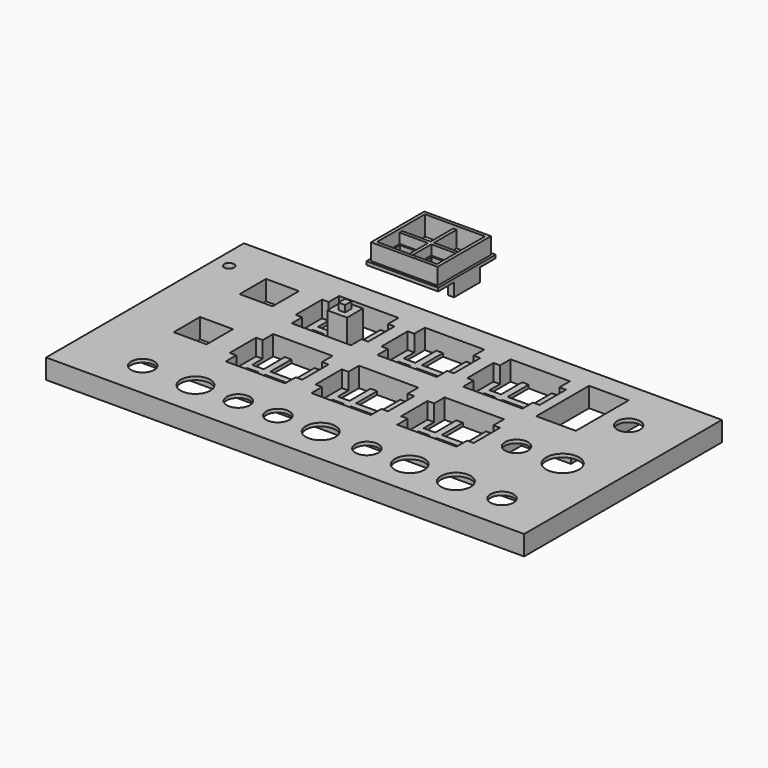
from build123d import *

# Parameters (mm, degrees)
F0_W      = 145
F0_H      = 75
F0_R      = 3.5
F0_R_2    = 4.5
F0_R_3    = 5
F0_R_4    = 1.5
F0_W_2    = 12
F0_H_2    = 20
F0_W_3    = 2
F0_H_3    = 10
F1_DEPTH  = 1
F2_DEPTH  = 5
F3_W      = 2
F3_H      = 10
F3_W_2    = 10
F4_DEPTH  = 5
F5_W      = 1.8
F5_H      = 9.8
F6_DEPTH  = 1
F7_DEPTH  = 4
F8_W      = 20.2
F8_H      = 20.2
F8_W_2    = 18.2
F8_H_2    = 18.2
F9_DEPTH  = 5
F11_W     = 6
F11_H     = 4
F11_H_2   = 2
F12_DEPTH = 8
F10_W     = 8.6
F10_H     = 1
F10_W_2   = 1
F10_H_2   = 8.6
F13_DEPTH = 6
F14_W     = 18.2
F14_H     = 18.2
F15_DEPTH = 1
F17_W     = 2
F17_H     = 2.5
F18_DEPTH = 2
F19_W     = 8.6
F19_H     = 8.6
F19_W_2   = 7.6
F19_H_2   = 7.6
F20_DEPTH = 2
F16_W     = 2
F16_H     = 2.5
F21_DEPTH = 2
F23_DEPTH = 5
F24_W     = 34
F24_H     = 2
F24_W_2   = 19
F25_DEPTH = 5


with BuildPart() as f1:
    # F0 (on Top) → F1 (new body)
    with BuildSketch(Plane.XY):
        with Locations((-82.504784634, -17.5405644029)):
            Rectangle(F0_W, F0_H)
        with Locations((-134.504784634, -44.0405644029)):
            Circle(F0_R, mode=Mode.SUBTRACT)
        with Locations((-118.504784634, -44.0405644029)):
            Circle(F0_R_2, mode=Mode.SUBTRACT)
        with Locations((-105.504784634, -44.0405644029)):
            Circle(F0_R, mode=Mode.SUBTRACT)
        with Locations((-93.504784634, -44.0405644029)):
            Circle(F0_R, mode=Mode.SUBTRACT)
        Polygon((-129.504784634, -16.0405644029), (-129.504784634, -26.0405644029), (-133.504784634, -26.0405644029), (-135.504784634, -26.0405644029), (-139.504784634, -26.0405644029), (-139.504784634, -16.0405644029), (-135.504784634, -16.0405644029), (-133.504784634, -16.0405644029), align=None, mode=Mode.SUBTRACT)
        Polygon((-102.504784634, -22.0405644029), (-102.504784634, -30.0405644029), (-105.9770819313, -30.0405644029), (-107.9770819313, -30.0405644029), (-114.9770819313, -30.0405644029), (-116.9770819313, -30.0405644029), (-120.504784634, -30.0405644029), (-120.504784634, -22.0405644029), (-120.504784634, -20.0405644029), (-120.504784634, -12.0405644029), (-116.9770819313, -12.0405644029), (-114.9770819313, -12.0405644029), (-107.9770819313, -12.0405644029), (-105.9770819313, -12.0405644029), (-102.504784634, -12.0405644029), (-102.504784634, -20.0405644029), align=None, mode=Mode.SUBTRACT)
        Polygon((-76.504784634, -12.0405644029), (-76.504784634, -20.0405644029), (-76.504784634, -22.0405644029), (-76.504784634, -30.0405644029), (-79.9770819313, -30.0405644029), (-81.9770819313, -30.0405644029), (-88.9770819313, -30.0405644029), (-90.9770819313, -30.0405644029), (-94.504784634, -30.0405644029), (-94.504784634, -22.0405644029), (-94.504784634, -20.0405644029), (-94.504784634, -12.0405644029), (-90.9770819313, -12.0405644029), (-88.9770819313, -12.0405644029), (-81.9770819313, -12.0405644029), (-79.9770819313, -12.0405644029), align=None, mode=Mode.SUBTRACT)
        with Locations((-80.504784634, -44.0405644029)):
            Circle(F0_R_2, mode=Mode.SUBTRACT)
        with Locations((-66.504784634, -44.0405644029)):
            Circle(F0_R, mode=Mode.SUBTRACT)
        with Locations((-53.504784634, -44.0405644029)):
            Circle(F0_R_2, mode=Mode.SUBTRACT)
        with Locations((-39.504784634, -44.0405644029)):
            Circle(F0_R_2, mode=Mode.SUBTRACT)
        with Locations((-25.504784634, -44.0405644029)):
            Circle(F0_R, mode=Mode.SUBTRACT)
        Polygon((-50.504784634, -12.0405644029), (-50.504784634, -20.0405644029), (-50.504784634, -22.0405644029), (-50.504784634, -30.0405644029), (-53.9770819313, -30.0405644029), (-55.9770819313, -30.0405644029), (-62.9770819313, -30.0405644029), (-64.9770819313, -30.0405644029), (-68.504784634, -30.0405644029), (-68.504784634, -22.0405644029), (-68.504784634, -20.0405644029), (-68.504784634, -12.0405644029), (-64.9770819313, -12.0405644029), (-62.9770819313, -12.0405644029), (-55.9770819313, -12.0405644029), (-53.9770819313, -12.0405644029), align=None, mode=Mode.SUBTRACT)
        with Locations((-39.504784634, -21.0405644029)):
            Circle(F0_R, mode=Mode.SUBTRACT)
        with Locations((-25.504784634, -21.0405644029)):
            Circle(F0_R_3, mode=Mode.SUBTRACT)
        with Locations((-150.504784634, 8.7571097538)):
            Circle(F0_R_4, mode=Mode.SUBTRACT)
        Polygon((-129.504784634, 8.9594355971), (-129.504784634, -1.0405644029), (-133.504784634, -1.0405644029), (-135.504784634, -1.0405644029), (-139.504784634, -1.0405644029), (-139.504784634, 8.9594355971), (-135.504784634, 8.9594355971), (-133.504784634, 8.9594355971), align=None, mode=Mode.SUBTRACT)
        Polygon((-102.504784634, 2.9594355971), (-102.504784634, -5.0405644029), (-106.004784634, -5.0405644029), (-108.004784634, -5.0405644029), (-115.004784634, -5.0405644029), (-117.004784634, -5.0405644029), (-120.504784634, -5.0405644029), (-120.504784634, 2.9594355971), (-120.504784634, 4.9594355971), (-120.504784634, 12.9594355971), (-117.004784634, 12.9594355971), (-115.004784634, 12.9594355971), (-108.004784634, 12.9594355971), (-106.004784634, 12.9594355971), (-102.504784634, 12.9594355971), (-102.504784634, 4.9594355971), align=None, mode=Mode.SUBTRACT)
        Polygon((-94.504784634, 12.9594355971), (-91.004784634, 12.9594355971), (-89.004784634, 12.9594355971), (-82.004784634, 12.9594355971), (-80.004784634, 12.9594355971), (-76.504784634, 12.9594355971), (-76.504784634, 4.9594355971), (-76.504784634, 2.9594355971), (-76.504784634, -5.0405644029), (-80.004784634, -5.0405644029), (-82.004784634, -5.0405644029), (-89.004784634, -5.0405644029), (-91.004784634, -5.0405644029), (-94.504784634, -5.0405644029), (-94.504784634, 2.9594355971), (-94.504784634, 4.9594355971), align=None, mode=Mode.SUBTRACT)
        Polygon((-68.504784634, 12.9594355971), (-65.004784634, 12.9594355971), (-63.004784634, 12.9594355971), (-56.004784634, 12.9594355971), (-54.004784634, 12.9594355971), (-50.504784634, 12.9594355971), (-50.504784634, 4.9594355971), (-50.504784634, 2.9594355971), (-50.504784634, -5.0405644029), (-54.004784634, -5.0405644029), (-56.004784634, -5.0405644029), (-63.004784634, -5.0405644029), (-65.004784634, -5.0405644029), (-68.504784634, -5.0405644029), (-68.504784634, 2.9594355971), (-68.504784634, 4.9594355971), align=None, mode=Mode.SUBTRACT)
        with Locations((-39.504784634, 3.9594355971)):
            Rectangle(F0_W_2, F0_H_2, mode=Mode.SUBTRACT)
        with Locations((-25.504784634, 3.9594355971)):
            Circle(F0_R, mode=Mode.SUBTRACT)
        Polygon((-108.004784634, -5.0405644029), (-106.004784634, -5.0405644029), (-106.004784634, 2.9594355971), (-102.504784634, 2.9594355971), (-102.504784634, 4.9594355971), (-106.004784634, 4.9594355971), (-106.004784634, 12.9594355971), (-108.004784634, 12.9594355971), (-108.004784634, 4.9594355971), (-115.004784634, 4.9594355971), (-115.004784634, 12.9594355971), (-117.004784634, 12.9594355971), (-117.004784634, 4.9594355971), (-120.504784634, 4.9594355971), (-120.504784634, 2.9594355971), (-117.004784634, 2.9594355971), (-117.004784634, -5.0405644029), (-115.004784634, -5.0405644029), (-115.004784634, 2.9594355971), (-108.004784634, 2.9594355971), align=None)
        Polygon((-107.9770819313, -30.0405644029), (-105.9770819313, -30.0405644029), (-105.9770819313, -22.0405644029), (-102.504784634, -22.0405644029), (-102.504784634, -20.0405644029), (-105.9770819313, -20.0405644029), (-105.9770819313, -12.0405644029), (-107.9770819313, -12.0405644029), (-107.9770819313, -20.0405644029), (-114.9770819313, -20.0405644029), (-114.9770819313, -12.0405644029), (-116.9770819313, -12.0405644029), (-116.9770819313, -20.0405644029), (-120.504784634, -20.0405644029), (-120.504784634, -22.0405644029), (-116.9770819313, -22.0405644029), (-116.9770819313, -30.0405644029), (-114.9770819313, -30.0405644029), (-114.9770819313, -22.0405644029), (-107.9770819313, -22.0405644029), align=None)
        Polygon((-91.004784634, 12.9594355971), (-91.004784634, 4.9594355971), (-94.504784634, 4.9594355971), (-94.504784634, 2.9594355971), (-91.004784634, 2.9594355971), (-91.004784634, -5.0405644029), (-89.004784634, -5.0405644029), (-89.004784634, 2.9594355971), (-82.004784634, 2.9594355971), (-82.004784634, -5.0405644029), (-80.004784634, -5.0405644029), (-80.004784634, 2.9594355971), (-76.504784634, 2.9594355971), (-76.504784634, 4.9594355971), (-80.004784634, 4.9594355971), (-80.004784634, 12.9594355971), (-82.004784634, 12.9594355971), (-82.004784634, 4.9594355971), (-89.004784634, 4.9594355971), (-89.004784634, 12.9594355971), align=None)
        Polygon((-65.004784634, 12.9594355971), (-65.004784634, 4.9594355971), (-68.504784634, 4.9594355971), (-68.504784634, 2.9594355971), (-65.004784634, 2.9594355971), (-65.004784634, -5.0405644029), (-63.004784634, -5.0405644029), (-63.004784634, 2.9594355971), (-56.004784634, 2.9594355971), (-56.004784634, -5.0405644029), (-54.004784634, -5.0405644029), (-54.004784634, 2.9594355971), (-50.504784634, 2.9594355971), (-50.504784634, 4.9594355971), (-54.004784634, 4.9594355971), (-54.004784634, 12.9594355971), (-56.004784634, 12.9594355971), (-56.004784634, 4.9594355971), (-63.004784634, 4.9594355971), (-63.004784634, 12.9594355971), align=None)
        Polygon((-50.504784634, -22.0405644029), (-50.504784634, -20.0405644029), (-53.9770819313, -20.0405644029), (-53.9770819313, -12.0405644029), (-55.9770819313, -12.0405644029), (-55.9770819313, -20.0405644029), (-62.9770819313, -20.0405644029), (-62.9770819313, -12.0405644029), (-64.9770819313, -12.0405644029), (-64.9770819313, -20.0405644029), (-68.504784634, -20.0405644029), (-68.504784634, -22.0405644029), (-64.9770819313, -22.0405644029), (-64.9770819313, -30.0405644029), (-62.9770819313, -30.0405644029), (-62.9770819313, -22.0405644029), (-55.9770819313, -22.0405644029), (-55.9770819313, -30.0405644029), (-53.9770819313, -30.0405644029), (-53.9770819313, -22.0405644029), align=None)
        Polygon((-76.504784634, -22.0405644029), (-76.504784634, -20.0405644029), (-79.9770819313, -20.0405644029), (-79.9770819313, -12.0405644029), (-81.9770819313, -12.0405644029), (-81.9770819313, -20.0405644029), (-88.9770819313, -20.0405644029), (-88.9770819313, -12.0405644029), (-90.9770819313, -12.0405644029), (-90.9770819313, -20.0405644029), (-94.504784634, -20.0405644029), (-94.504784634, -22.0405644029), (-90.9770819313, -22.0405644029), (-90.9770819313, -30.0405644029), (-88.9770819313, -30.0405644029), (-88.9770819313, -22.0405644029), (-81.9770819313, -22.0405644029), (-81.9770819313, -30.0405644029), (-79.9770819313, -30.0405644029), (-79.9770819313, -22.0405644029), align=None)
        with Locations((-134.504784634, 3.9594355971)):
            Rectangle(F0_W_3, F0_H_3)
        with Locations((-134.504784634, -21.0405644029)):
            Rectangle(F0_W_3, F0_H_3)
    extrude(amount=F1_DEPTH)

    # F2 (add): a face of the model
    f2_faces = [f1.faces().sort_by_distance(p)[0] for p in [
        (-82.504784634, 18.3269528253, 1),
    ]]
    extrude(f2_faces, amount=F2_DEPTH)

    # F3 (on face) → F4 (cut)
    with BuildSketch(Plane.XY.offset(6)):
        Polygon((-120.504784634, -5.0405644029), (-102.504784634, -5.0405644029), (-102.504784634, -1.0405644029), (-102.504784634, 8.9594355971), (-102.504784634, 12.9594355971), (-120.504784634, 12.9594355971), (-120.504784634, 8.9594355971), (-120.504784634, -1.0405644029), align=None)
        with Locations((-101.504784634, 3.9594355971)):
            Rectangle(F3_W, F3_H)
        with Locations((-121.504784634, 3.9594355971)):
            Rectangle(F3_W, F3_H)
        Polygon((-120.504784634, -30.0405644029), (-102.504784634, -30.0405644029), (-102.504784634, -26.0405644029), (-102.504784634, -16.0405644029), (-102.504784634, -12.0405644029), (-120.504784634, -12.0405644029), (-120.504784634, -16.0405644029), (-120.504784634, -26.0405644029), align=None)
        with Locations((-101.504784634, -21.0405644029)):
            Rectangle(F3_W, F3_H)
        with Locations((-121.504784634, -21.0405644029)):
            Rectangle(F3_W, F3_H)
        with Locations((-75.504784634, 3.9594355971)):
            Rectangle(F3_W, F3_H)
        Polygon((-76.504784634, -5.0405644029), (-76.504784634, -1.0405644029), (-76.504784634, 8.9594355971), (-76.504784634, 12.9594355971), (-94.504784634, 12.9594355971), (-94.504784634, 8.9594355971), (-94.504784634, -1.0405644029), (-94.504784634, -5.0405644029), align=None)
        with Locations((-95.504784634, 3.9594355971)):
            Rectangle(F3_W, F3_H)
        with Locations((-49.504784634, 3.9594355971)):
            Rectangle(F3_W, F3_H)
        Polygon((-50.504784634, -5.0405644029), (-50.504784634, -1.0405644029), (-50.504784634, 8.9594355971), (-50.504784634, 12.9594355971), (-68.504784634, 12.9594355971), (-68.504784634, 8.9594355971), (-68.504784634, -1.0405644029), (-68.504784634, -5.0405644029), align=None)
        with Locations((-69.504784634, 3.9594355971)):
            Rectangle(F3_W, F3_H)
        with Locations((-75.504784634, -21.0405644029)):
            Rectangle(F3_W, F3_H)
        Polygon((-76.504784634, -26.0405644029), (-76.504784634, -16.0405644029), (-76.504784634, -12.0405644029), (-94.504784634, -12.0405644029), (-94.504784634, -16.0405644029), (-94.504784634, -26.0405644029), (-94.504784634, -30.0405644029), (-76.504784634, -30.0405644029), align=None)
        with Locations((-95.504784634, -21.0405644029)):
            Rectangle(F3_W, F3_H)
        with Locations((-49.504784634, -21.0405644029)):
            Rectangle(F3_W, F3_H)
        Polygon((-50.504784634, -26.0405644029), (-50.504784634, -16.0405644029), (-50.504784634, -12.0405644029), (-68.504784634, -12.0405644029), (-68.504784634, -16.0405644029), (-68.504784634, -26.0405644029), (-68.504784634, -30.0405644029), (-50.504784634, -30.0405644029), align=None)
        with Locations((-69.504784634, -21.0405644029)):
            Rectangle(F3_W, F3_H)
        with Locations((-134.504784634, 3.9594355971)):
            Rectangle(F3_W_2, F3_H)
        with Locations((-134.504784634, -21.0405644029)):
            Rectangle(F3_W_2, F3_H)
    extrude(amount=-F4_DEPTH, mode=Mode.SUBTRACT)

    # F11 (on face) → F12 (join)
    with BuildSketch(Plane.XY.offset(1)):
        with Locations((-111.504784634, 4.9594355971)):
            Rectangle(F11_W, F11_H)
        with Locations((-111.504784634, 1.9594355971)):
            Rectangle(F11_W, F11_H_2)
    extrude(amount=F12_DEPTH)

    # F17 (on face) → F18 (join)
    with BuildSketch(Plane.XY.offset(9)):
        with Locations((-111.504784634, 3.9594355971)):
            Rectangle(F17_W, F17_H)
    extrude(amount=F18_DEPTH)

    # F22 (on face) → F23 (cut)
    with BuildSketch(Plane.XY):
        Polygon((-155.004784634, -34.0405644029), (-155.004784634, -55.0405644029), (-46.004784634, -55.0405644029), (-10.004784634, -55.0405644029), (-10.004784634, -34.0405644029), (-10.004784634, -11.0405644029), (-10.004784634, 19.9594355971), (-31.004784634, 19.9594355971), (-31.004784634, -11.0405644029), (-46.004784634, -11.0405644029), (-46.004784634, -34.0405644029), align=None)
    extrude(amount=F23_DEPTH, mode=Mode.SUBTRACT)

    # F24 (on face) → F25 (join)
    with BuildSketch(Plane(origin=(0, 0, 5), x_dir=(1, 0, 0), z_dir=(0, 0, -1))):
        Polygon((-153.004784634, 55.0405644029), (-155.004784634, 55.0405644029), (-155.004784634, 34.0405644029), (-153.004784634, 34.0405644029), (-153.004784634, 53.0405644029), align=None)
        Polygon((-10.004784634, 55.0405644029), (-153.004784634, 55.0405644029), (-153.004784634, 53.0405644029), (-12.004784634, 53.0405644029), (-10.004784634, 53.0405644029), align=None)
        Polygon((-10.004784634, 53.0405644029), (-12.004784634, 53.0405644029), (-12.004784634, 34.0405644029), (-12.004784634, 32.0405644029), (-12.004784634, -17.9594355971), (-12.004784634, -19.9594355971), (-10.004784634, -19.9594355971), align=None)
        with Locations((-29.004784634, 33.0405644029)):
            Rectangle(F24_W, F24_H)
        with Locations((-21.504784634, -18.9594355971)):
            Rectangle(F24_W_2, F24_H)
    extrude(amount=F25_DEPTH)


with BuildPart() as f6:
    # F5 (on Top) → F6 (new body)
    with BuildSketch(Plane.XY):
        Polygon((-132.6183355093, 38.3936729491), (-110.8183355093, 38.3936729491), (-110.8183355093, 44.3936729491), (-112.6183355093, 44.3936729491), (-112.6183355093, 40.1936729491), (-130.8183355093, 40.1936729491), (-130.8183355093, 44.3936729491), (-132.6183355093, 44.3936729491), align=None)
        with Locations((-111.7183355093, 49.2936729491)):
            Rectangle(F5_W, F5_H)
        with Locations((-131.7183355093, 49.2936729491)):
            Rectangle(F5_W, F5_H)
        Polygon((-112.6183355093, 54.1936729491), (-110.8183355093, 54.1936729491), (-110.8183355093, 60.1936729491), (-132.6183355093, 60.1936729491), (-132.6183355093, 54.1936729491), (-130.8183355093, 54.1936729491), (-130.8183355093, 58.3936729491), (-112.6183355093, 58.3936729491), align=None)
    extrude(amount=F6_DEPTH)

    # F5 (on Top) → F7 (join)
    with BuildSketch(Plane.XY):
        with Locations((-131.7183355093, 49.2936729491)):
            Rectangle(F5_W, F5_H)
        with Locations((-111.7183355093, 49.2936729491)):
            Rectangle(F5_W, F5_H)
    extrude(amount=-F7_DEPTH)

    # F8 (on face) → F9 (join)
    with BuildSketch(Plane.XY.offset(1)):
        with Locations((-121.7183355093, 49.2936729491)):
            Rectangle(F8_W, F8_H)
        with Locations((-121.7183355093, 49.2936729491)):
            Rectangle(F8_W_2, F8_H_2, mode=Mode.SUBTRACT)
    extrude(amount=F9_DEPTH)

    # F10 (on face) → F13 (join)
    with BuildSketch(Plane.XY.offset(6)):
        with Locations((-116.9183355093, 49.2936729491)):
            Rectangle(F10_W, F10_H)
        with Locations((-121.7183355093, 44.4936729491)):
            Rectangle(F10_W_2, F10_H_2)
        with Locations((-121.7183355093, 49.2936729491)):
            Rectangle(F10_W_2, F10_H)
        with Locations((-126.5183355093, 49.2936729491)):
            Rectangle(F10_W, F10_H)
        with Locations((-121.7183355093, 54.0936729491)):
            Rectangle(F10_W_2, F10_H_2)
    extrude(amount=-F13_DEPTH)

    # F14 (on face) → F15 (cut)
    with BuildSketch(Plane.XY.offset(6)):
        with Locations((-121.7183355093, 49.2936729491)):
            Rectangle(F14_W, F14_H)
    extrude(amount=-F15_DEPTH, mode=Mode.SUBTRACT)

    # F19 (on face) → F20 (join)
    with BuildSketch(Plane(origin=(0, 0, 0), x_dir=(1, 0, 0), z_dir=(0, 0, -1))):
        with Locations((-126.5183355093, -44.4936729491)):
            Rectangle(F19_W, F19_H)
        with Locations((-126.5183355093, -44.4936729491)):
            Rectangle(F19_W_2, F19_H_2, mode=Mode.SUBTRACT)
        with Locations((-116.9183355093, -44.4936729491)):
            Rectangle(F19_W, F19_H)
        with Locations((-116.9183355093, -44.4936729491)):
            Rectangle(F19_W_2, F19_H_2, mode=Mode.SUBTRACT)
    extrude(amount=-F20_DEPTH)

    # F16 (on face) → F21 (cut)
    with BuildSketch(Plane(origin=(0, 0, 0), x_dir=(1, 0, 0), z_dir=(0, 0, -1))):
        with Locations((-121.7183355093, -49.2936729491)):
            Rectangle(F16_W, F16_H)
    extrude(amount=-F21_DEPTH, mode=Mode.SUBTRACT)


solid = Compound([f1.part, f6.part])
